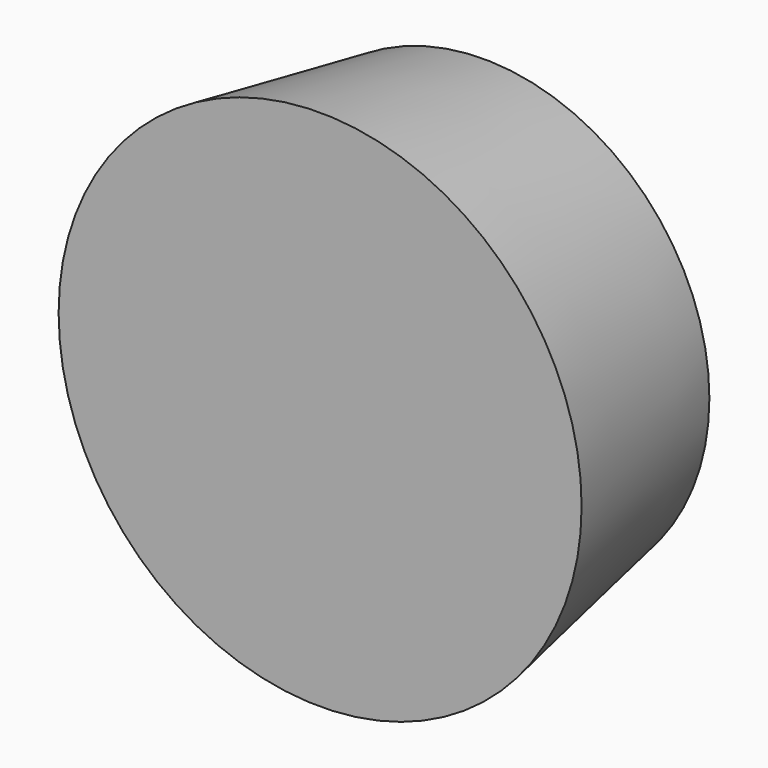
from build123d import *

# Parameters (mm, degrees)
F0_R     = 11
F1_DEPTH = 10
F1_TAPER = -10


# Not quite as in the source:
# - the program builds the solid bodies; features that only make, move or delete a surface that nothing else refers to are left out


with BuildPart() as f1:
    # F0 (on Front) → F1 (new body)
    with BuildSketch(Plane.XZ):
        Circle(F0_R)
    extrude(amount=F1_DEPTH, taper=F1_TAPER)


solid = f1.part
